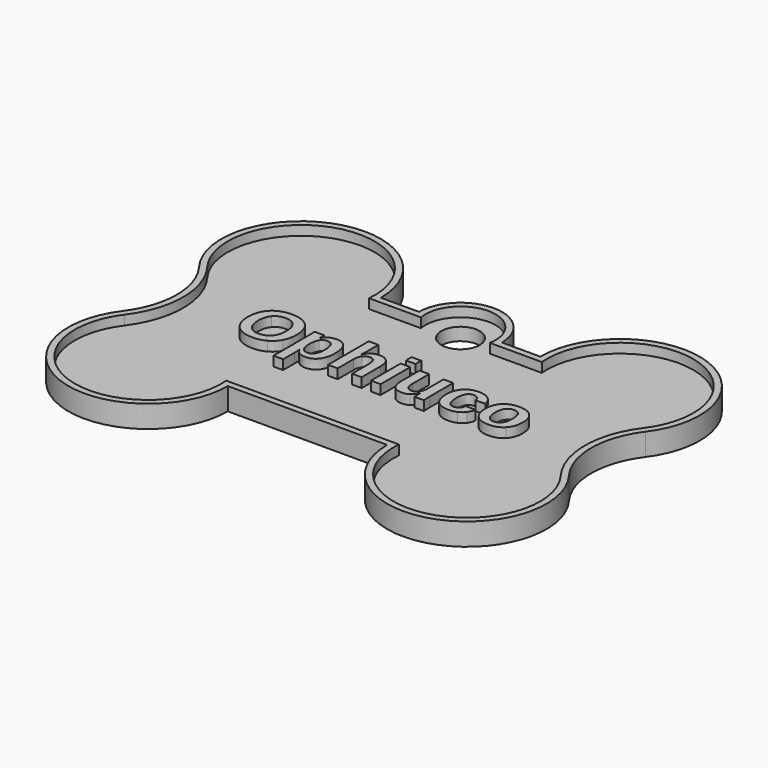
from build123d import *

# Parameters (mm, degrees)
F0_R     = 3
F1_DEPTH = 3.5
F2_W     = 1.5111876076
F2_H     = 5.8192771084
F2_H_2   = 1.1135972461
F3_DEPTH = 1.5


with BuildPart() as f1:
    # F0 (on Top) → F1 (new body)
    with BuildSketch(Plane.XY):
        with BuildLine():
            Line((28.5, 30), (22.5, 30))
            ThreePointArc((22.5, 30), (6.0471529248, 41.8585412256), (0, 22.5))
            ThreePointArc((0, 22.5), (2.5, 15), (0, 7.5))
            ThreePointArc((0, 7.5), (6.0471529248, -11.8585412256), (22.5, 0))
            Line((22.5, 0), (47.5, 0))
            ThreePointArc((47.5, 0), (63.9528470752, -11.8585412256), (70, 7.5))
            ThreePointArc((70, 7.5), (67.5, 15), (70, 22.5))
            ThreePointArc((70, 22.5), (63.9528470752, 41.8585412256), (47.5, 30))
            Line((47.5, 30), (41.5, 30))
            ThreePointArc((41.5, 30), (35, 36.5), (28.5, 30))
        make_face()
        with Locations((35, 30)):
            Circle(F0_R, mode=Mode.SUBTRACT)
    extrude(amount=F1_DEPTH)

    # F2 (on face) → F3 (cut)
    with BuildSketch(Plane.XY.offset(3.5)):
        with BuildLine():
            Line((21.4564392374, 1), (48.5435607626, 1))
            ThreePointArc((48.5435607626, 1), (63.1583824195, -11.0577855148), (69.2, 6.9))
            ThreePointArc((69.2, 6.9), (66.5, 15), (69.2, 23.1))
            ThreePointArc((69.2, 23.1), (63.1583824195, 41.0577855148), (48.5435607626, 29))
            Line((48.5435607626, 29), (40.4083269132, 29))
            ThreePointArc((40.4083269132, 29), (35, 35.5), (29.5916730868, 29))
            Line((29.5916730868, 29), (21.4564392374, 29))
            ThreePointArc((21.4564392374, 29), (6.8416175805, 41.0577855148), (0.8, 23.1))
            ThreePointArc((0.8, 23.1), (3.5, 15), (0.8, 6.9))
            ThreePointArc((0.8, 6.9), (6.8416175805, -11.0577855148), (21.4564392374, 1))
        make_face()
        with BuildLine():
            add(Edge.make_bspline(
                [(26.7857142857, 17.2297762478), (27.3450946644, 16.4475043029), (27.3450946644, 15.0051635112)],
                knots=[0, 0, 0, 1, 1, 1], degree=2))
            add(Edge.make_bspline(
                [(27.3450946644, 15.0051635112), (27.3450946644, 13.5473321859), (26.7616179002, 12.7538726334)],
                knots=[0, 0, 0, 1, 1, 1], degree=2))
            add(Edge.make_bspline(
                [(26.7616179002, 12.7538726334), (26.178141136, 11.9604130809), (25.1127366609, 11.9604130809)],
                knots=[0, 0, 0, 1, 1, 1], degree=2))
            add(Edge.make_bspline(
                [(25.1127366609, 11.9604130809), (24.5, 11.9604130809), (24.0456110155, 12.2271944923)],
                knots=[0, 0, 0, 1, 1, 1], degree=2))
            add(Edge.make_bspline(
                [(24.0456110155, 12.2271944923), (23.591222031, 12.4939759036), (23.3485370052, 12.9948364888)],
                knots=[0, 0, 0, 1, 1, 1], degree=2))
            Line((23.3485370052, 12.9948364888), (23.3158347676, 12.9948364888))
            add(Edge.make_bspline(
                [(23.3158347676, 12.9948364888), (23.3485370052, 12.8330464716), (23.3485370052, 12.0154905336)],
                knots=[0, 0, 0, 1, 1, 1], degree=2))
            Line((23.3485370052, 12.0154905336), (23.3485370052, 9.7831325301))
            Line((23.3485370052, 9.7831325301), (21.8373493976, 9.7831325301))
            Line((21.8373493976, 9.7831325301), (21.8373493976, 16.5490533563))
            add(Edge.make_bspline(
                [(21.8373493976, 16.5490533563), (21.8373493976, 17.3717728055), (21.7943201377, 17.8881239243)],
                knots=[0, 0, 0, 1, 1, 1], degree=2))
            Line((21.7943201377, 17.8881239243), (23.2624784854, 17.8881239243))
            add(Edge.make_bspline(
                [(23.2624784854, 17.8881239243), (23.2900172117, 17.7917383821), (23.3089500861, 17.5068846816)],
                knots=[0, 0, 0, 1, 1, 1], degree=2))
            add(Edge.make_bspline(
                [(23.3089500861, 17.5068846816), (23.3278829604, 17.2220309811), (23.3278829604, 16.9414802065)],
                knots=[0, 0, 0, 1, 1, 1], degree=2))
            Line((23.3278829604, 16.9414802065), (23.3485370052, 16.9414802065))
            add(Edge.make_bspline(
                [(23.3485370052, 16.9414802065), (23.8597246127, 18.0120481928), (25.2091222031, 18.0120481928)],
                knots=[0, 0, 0, 1, 1, 1], degree=2))
            add(Edge.make_bspline(
                [(25.2091222031, 18.0120481928), (26.2263339071, 18.0120481928), (26.7857142857, 17.2297762478)],
                knots=[0, 0, 0, 1, 1, 1], degree=2))
        make_face(mode=Mode.SUBTRACT)
        with Locations((36.0490533563, 14.9784853701)):
            Rectangle(F2_W, F2_H, mode=Mode.SUBTRACT)
        with BuildLine():
            Line((38.2676419966, 17.8881239243), (39.7788296041, 17.8881239243))
            Line((39.7788296041, 17.8881239243), (39.7788296041, 14.6230636833))
            add(Edge.make_bspline(
                [(39.7788296041, 14.6230636833), (39.7788296041, 13.091222031), (40.8115318417, 13.091222031)],
                knots=[0, 0, 0, 1, 1, 1], degree=2))
            add(Edge.make_bspline(
                [(40.8115318417, 13.091222031), (41.3605851979, 13.091222031), (41.6962134251, 13.5619621343)],
                knots=[0, 0, 0, 1, 1, 1], degree=2))
            add(Edge.make_bspline(
                [(41.6962134251, 13.5619621343), (42.0318416523, 14.0327022375), (42.0318416523, 14.769363167)],
                knots=[0, 0, 0, 1, 1, 1], degree=2))
            Line((42.0318416523, 14.769363167), (42.0318416523, 17.8881239243))
            Line((42.0318416523, 17.8881239243), (43.5447504303, 17.8881239243))
            Line((43.5447504303, 17.8881239243), (43.5447504303, 13.3700516351))
            add(Edge.make_bspline(
                [(43.5447504303, 13.3700516351), (43.5447504303, 12.6282271945), (43.5877796902, 12.0688468158)],
                knots=[0, 0, 0, 1, 1, 1], degree=2))
            Line((43.5877796902, 12.0688468158), (42.1454388985, 12.0688468158))
            add(Edge.make_bspline(
                [(42.1454388985, 12.0688468158), (42.0817555938, 12.843373494), (42.0817555938, 13.2254733219)],
                knots=[0, 0, 0, 1, 1, 1], degree=2))
            Line((42.0817555938, 13.2254733219), (42.0542168675, 13.2254733219))
            add(Edge.make_bspline(
                [(42.0542168675, 13.2254733219), (41.7530120482, 12.5645438898), (41.2874354561, 12.2624784854)],
                knots=[0, 0, 0, 1, 1, 1], degree=2))
            add(Edge.make_bspline(
                [(41.2874354561, 12.2624784854), (40.821858864, 11.9604130809), (40.1815834768, 11.9604130809)],
                knots=[0, 0, 0, 1, 1, 1], degree=2))
            add(Edge.make_bspline(
                [(40.1815834768, 11.9604130809), (39.2573149742, 11.9604130809), (38.7624784854, 12.5283993115)],
                knots=[0, 0, 0, 1, 1, 1], degree=2))
            add(Edge.make_bspline(
                [(38.7624784854, 12.5283993115), (38.2676419966, 13.0963855422), (38.2676419966, 14.1927710843)],
                knots=[0, 0, 0, 1, 1, 1], degree=2))
            Line((38.2676419966, 14.1927710843), (38.2676419966, 17.8881239243))
        make_face(mode=Mode.SUBTRACT)
        with BuildLine():
            add(Edge.make_bspline(
                [(48.7771084337, 12.2160068847), (48.2125645439, 11.9604130809), (47.5068846816, 11.9604130809)],
                knots=[0, 0, 0, 1, 1, 1], degree=2))
            add(Edge.make_bspline(
                [(47.5068846816, 11.9604130809), (46.1850258176, 11.9604130809), (45.4638554217, 12.7487091222)],
                knots=[0, 0, 0, 1, 1, 1], degree=2))
            add(Edge.make_bspline(
                [(45.4638554217, 12.7487091222), (44.7426850258, 13.5370051635), (44.7426850258, 14.9466437177)],
                knots=[0, 0, 0, 1, 1, 1], degree=2))
            add(Edge.make_bspline(
                [(44.7426850258, 14.9466437177), (44.7426850258, 16.3872633391), (45.4690189329, 17.1919104991)],
                knots=[0, 0, 0, 1, 1, 1], degree=2))
            add(Edge.make_bspline(
                [(45.4690189329, 17.1919104991), (46.1953528399, 17.9965576592), (47.5292598967, 17.9965576592)],
                knots=[0, 0, 0, 1, 1, 1], degree=2))
            add(Edge.make_bspline(
                [(47.5292598967, 17.9965576592), (48.5567986231, 17.9965576592), (49.2289156627, 17.4802065404)],
                knots=[0, 0, 0, 1, 1, 1], degree=2))
            add(Edge.make_bspline(
                [(49.2289156627, 17.4802065404), (49.9010327022, 16.9638554217), (50.0731497418, 16.0550774527)],
                knots=[0, 0, 0, 1, 1, 1], degree=2))
            Line((50.0731497418, 16.0550774527), (48.5516351119, 15.9793459552))
            add(Edge.make_bspline(
                [(48.5516351119, 15.9793459552), (48.4862306368, 16.4251290878), (48.2280550775, 16.6919104991)],
                knots=[0, 0, 0, 1, 1, 1], degree=2))
            add(Edge.make_bspline(
                [(48.2280550775, 16.6919104991), (47.9698795181, 16.9586919105), (47.4965576592, 16.9586919105)],
                knots=[0, 0, 0, 1, 1, 1], degree=2))
            add(Edge.make_bspline(
                [(47.4965576592, 16.9586919105), (46.3296041308, 16.9586919105), (46.3296041308, 15.0051635112)],
                knots=[0, 0, 0, 1, 1, 1], degree=2))
            add(Edge.make_bspline(
                [(46.3296041308, 15.0051635112), (46.3296041308, 12.9948364888), (47.5189328744, 12.9948364888)],
                knots=[0, 0, 0, 1, 1, 1], degree=2))
            add(Edge.make_bspline(
                [(47.5189328744, 12.9948364888), (47.9492254733, 12.9948364888), (48.239242685, 13.2659208262)],
                knots=[0, 0, 0, 1, 1, 1], degree=2))
            add(Edge.make_bspline(
                [(48.239242685, 13.2659208262), (48.5292598967, 13.5370051635), (48.599827883, 14.0757314974)],
                knots=[0, 0, 0, 1, 1, 1], degree=2))
            Line((48.599827883, 14.0757314974), (50.1161790017, 14.0051635112))
            add(Edge.make_bspline(
                [(50.1161790017, 14.0051635112), (50.0352839931, 13.4079173838), (49.6884681583, 12.9397590361)],
                knots=[0, 0, 0, 1, 1, 1], degree=2))
            add(Edge.make_bspline(
                [(49.6884681583, 12.9397590361), (49.3416523236, 12.4716006885), (48.7771084337, 12.2160068847)],
                knots=[0, 0, 0, 1, 1, 1], degree=2))
        make_face(mode=Mode.SUBTRACT)
        with BuildLine():
            add(Edge.make_bspline(
                [(55.9862306368, 17.2194492255), (56.7358003442, 16.4423407917), (56.7358003442, 14.9845094664)],
                knots=[0, 0, 0, 1, 1, 1], degree=2))
            add(Edge.make_bspline(
                [(56.7358003442, 14.9845094664), (56.7358003442, 13.569707401), (55.9509466437, 12.765060241)],
                knots=[0, 0, 0, 1, 1, 1], degree=2))
            add(Edge.make_bspline(
                [(55.9509466437, 12.765060241), (55.1660929432, 11.9604130809), (53.7788296041, 11.9604130809)],
                knots=[0, 0, 0, 1, 1, 1], degree=2))
            add(Edge.make_bspline(
                [(53.7788296041, 11.9604130809), (52.417383821, 11.9604130809), (51.6428571429, 12.7676419966)],
                knots=[0, 0, 0, 1, 1, 1], degree=2))
            add(Edge.make_bspline(
                [(51.6428571429, 12.7676419966), (50.8683304647, 13.5748709122), (50.8683304647, 14.9845094664)],
                knots=[0, 0, 0, 1, 1, 1], degree=2))
            add(Edge.make_bspline(
                [(50.8683304647, 14.9845094664), (50.8683304647, 16.3872633391), (51.6428571429, 17.1919104991)],
                knots=[0, 0, 0, 1, 1, 1], degree=2))
            add(Edge.make_bspline(
                [(51.6428571429, 17.1919104991), (52.417383821, 17.9965576592), (53.8098106713, 17.9965576592)],
                knots=[0, 0, 0, 1, 1, 1], degree=2))
            add(Edge.make_bspline(
                [(53.8098106713, 17.9965576592), (55.2366609294, 17.9965576592), (55.9862306368, 17.2194492255)],
                knots=[0, 0, 0, 1, 1, 1], degree=2))
        make_face(mode=Mode.SUBTRACT)
        with BuildLine():
            add(Edge.make_bspline(
                [(19.591222031, 18.7280550775), (20.6049913941, 17.6953528399), (20.6049913941, 15.8932874355)],
                knots=[0, 0, 0, 1, 1, 1], degree=2))
            add(Edge.make_bspline(
                [(20.6049913941, 15.8932874355), (20.6049913941, 14.7091222031), (20.1376936317, 13.8115318417)],
                knots=[0, 0, 0, 1, 1, 1], degree=2))
            add(Edge.make_bspline(
                [(20.1376936317, 13.8115318417), (19.6703958692, 12.9139414802), (18.7986230637, 12.4371772806)],
                knots=[0, 0, 0, 1, 1, 1], degree=2))
            add(Edge.make_bspline(
                [(18.7986230637, 12.4371772806), (17.9268502582, 11.9604130809), (16.765060241, 11.9604130809)],
                knots=[0, 0, 0, 1, 1, 1], degree=2))
            add(Edge.make_bspline(
                [(16.765060241, 11.9604130809), (14.9802065404, 11.9604130809), (13.9664371773, 13.0120481928)],
                knots=[0, 0, 0, 1, 1, 1], degree=2))
            add(Edge.make_bspline(
                [(13.9664371773, 13.0120481928), (12.9526678141, 14.0636833046), (12.9526678141, 15.8932874355)],
                knots=[0, 0, 0, 1, 1, 1], degree=2))
            add(Edge.make_bspline(
                [(12.9526678141, 15.8932874355), (12.9526678141, 17.7160068847), (13.9638554217, 18.7383820998)],
                knots=[0, 0, 0, 1, 1, 1], degree=2))
            add(Edge.make_bspline(
                [(13.9638554217, 18.7383820998), (14.9750430293, 19.760757315), (16.7762478485, 19.760757315)],
                knots=[0, 0, 0, 1, 1, 1], degree=2))
            add(Edge.make_bspline(
                [(16.7762478485, 19.760757315), (18.5774526678, 19.760757315), (19.591222031, 18.7280550775)],
                knots=[0, 0, 0, 1, 1, 1], degree=2))
        make_face(mode=Mode.SUBTRACT)
        with BuildLine():
            Line((30.0335628227, 16.7263339071), (30.0559380379, 16.7263339071))
            add(Edge.make_bspline(
                [(30.0559380379, 16.7263339071), (30.3623063683, 17.3941480207), (30.8244406196, 17.6953528399)],
                knots=[0, 0, 0, 1, 1, 1], degree=2))
            add(Edge.make_bspline(
                [(30.8244406196, 17.6953528399), (31.2865748709, 17.9965576592), (31.9268502582, 17.9965576592)],
                knots=[0, 0, 0, 1, 1, 1], degree=2))
            add(Edge.make_bspline(
                [(31.9268502582, 17.9965576592), (32.8528399312, 17.9965576592), (33.34767642, 17.425989673)],
                knots=[0, 0, 0, 1, 1, 1], degree=2))
            add(Edge.make_bspline(
                [(33.34767642, 17.425989673), (33.8425129088, 16.8554216867), (33.8425129088, 15.7590361446)],
                knots=[0, 0, 0, 1, 1, 1], degree=2))
            Line((33.8425129088, 15.7590361446), (33.8425129088, 12.0688468158))
            Line((33.8425129088, 12.0688468158), (32.3364888124, 12.0688468158))
            Line((32.3364888124, 12.0688468158), (32.3364888124, 15.3287435456))
            add(Edge.make_bspline(
                [(32.3364888124, 15.3287435456), (32.3364888124, 16.8605851979), (31.2969018933, 16.8605851979)],
                knots=[0, 0, 0, 1, 1, 1], degree=2))
            add(Edge.make_bspline(
                [(31.2969018933, 16.8605851979), (30.7495697074, 16.8605851979), (30.413080895, 16.3907056799)],
                knots=[0, 0, 0, 1, 1, 1], degree=2))
            add(Edge.make_bspline(
                [(30.413080895, 16.3907056799), (30.0765920826, 15.9208261618), (30.0765920826, 15.182444062)],
                knots=[0, 0, 0, 1, 1, 1], degree=2))
            Line((30.0765920826, 15.182444062), (30.0765920826, 12.0688468158))
            Line((30.0765920826, 12.0688468158), (28.565404475, 12.0688468158))
            Line((28.565404475, 12.0688468158), (28.565404475, 20.0516351119))
            Line((28.565404475, 20.0516351119), (30.0765920826, 20.0516351119))
            Line((30.0765920826, 20.0516351119), (30.0765920826, 17.8726333907))
            add(Edge.make_bspline(
                [(30.0765920826, 17.8726333907), (30.0765920826, 17.2857142857), (30.0335628227, 16.7263339071)],
                knots=[0, 0, 0, 1, 1, 1], degree=2))
        make_face(mode=Mode.SUBTRACT)
        with Locations((36.0490533563, 19.4948364888)):
            Rectangle(F2_W, F2_H_2, mode=Mode.SUBTRACT)
        with BuildLine():
            add(Edge.make_bspline(
                [(18.408777969, 13.908777969), (18.987091222, 14.6075731497), (18.987091222, 15.8932874355)],
                knots=[0, 0, 0, 1, 1, 1], degree=2))
            add(Edge.make_bspline(
                [(18.987091222, 15.8932874355), (18.987091222, 17.1187607573), (18.4061962134, 17.8158347676)],
                knots=[0, 0, 0, 1, 1, 1], degree=2))
            add(Edge.make_bspline(
                [(18.4061962134, 17.8158347676), (17.8253012048, 18.512908778), (16.7753872633, 18.512908778)],
                knots=[0, 0, 0, 1, 1, 1], degree=2))
            add(Edge.make_bspline(
                [(16.7753872633, 18.512908778), (15.7117039587, 18.512908778), (15.1308089501, 17.821858864)],
                knots=[0, 0, 0, 1, 1, 1], degree=2))
            add(Edge.make_bspline(
                [(15.1308089501, 17.821858864), (14.5499139415, 17.1308089501), (14.5499139415, 15.8932874355)],
                knots=[0, 0, 0, 1, 1, 1], degree=2))
            add(Edge.make_bspline(
                [(14.5499139415, 15.8932874355), (14.5499139415, 14.6454388985), (15.1437177281, 13.9277108434)],
                knots=[0, 0, 0, 1, 1, 1], degree=2))
            add(Edge.make_bspline(
                [(15.1437177281, 13.9277108434), (15.7375215146, 13.2099827883), (16.765060241, 13.2099827883)],
                knots=[0, 0, 0, 1, 1, 1], degree=2))
            add(Edge.make_bspline(
                [(16.765060241, 13.2099827883), (17.830464716, 13.2099827883), (18.408777969, 13.908777969)],
                knots=[0, 0, 0, 1, 1, 1], degree=2))
        make_face()
        with BuildLine():
            add(Edge.make_bspline(
                [(24.5585197935, 12.9948364888), (25.7685025818, 12.9948364888), (25.7685025818, 15.0051635112)],
                knots=[0, 0, 0, 1, 1, 1], degree=2))
            add(Edge.make_bspline(
                [(25.7685025818, 15.0051635112), (25.7685025818, 16.9638554217), (24.5688468158, 16.9638554217)],
                knots=[0, 0, 0, 1, 1, 1], degree=2))
            add(Edge.make_bspline(
                [(24.5688468158, 16.9638554217), (23.9664371773, 16.9638554217), (23.6471600688, 16.4363166954)],
                knots=[0, 0, 0, 1, 1, 1], degree=2))
            add(Edge.make_bspline(
                [(23.6471600688, 16.4363166954), (23.3278829604, 15.908777969), (23.3278829604, 14.9621342513)],
                knots=[0, 0, 0, 1, 1, 1], degree=2))
            add(Edge.make_bspline(
                [(23.3278829604, 14.9621342513), (23.3278829604, 14.0206540448), (23.6471600688, 13.5077452668)],
                knots=[0, 0, 0, 1, 1, 1], degree=2))
            add(Edge.make_bspline(
                [(23.6471600688, 13.5077452668), (23.9664371773, 12.9948364888), (24.5585197935, 12.9948364888)],
                knots=[0, 0, 0, 1, 1, 1], degree=2))
        make_face()
        with BuildLine():
            add(Edge.make_bspline(
                [(53.7616179002, 12.9948364888), (55.1557659208, 12.9948364888), (55.1557659208, 14.9845094664)],
                knots=[0, 0, 0, 1, 1, 1], degree=2))
            add(Edge.make_bspline(
                [(55.1557659208, 14.9845094664), (55.1557659208, 16.0223752151), (54.8166953528, 16.4905335628)],
                knots=[0, 0, 0, 1, 1, 1], degree=2))
            add(Edge.make_bspline(
                [(54.8166953528, 16.4905335628), (54.4776247849, 16.9586919105), (53.8321858864, 16.9586919105)],
                knots=[0, 0, 0, 1, 1, 1], degree=2))
            add(Edge.make_bspline(
                [(53.8321858864, 16.9586919105), (52.4552495697, 16.9586919105), (52.4552495697, 14.9845094664)],
                knots=[0, 0, 0, 1, 1, 1], degree=2))
            add(Edge.make_bspline(
                [(52.4552495697, 14.9845094664), (52.4552495697, 14.0103270224), (52.7917383821, 13.5025817556)],
                knots=[0, 0, 0, 1, 1, 1], degree=2))
            add(Edge.make_bspline(
                [(52.7917383821, 13.5025817556), (53.1282271945, 12.9948364888), (53.7616179002, 12.9948364888)],
                knots=[0, 0, 0, 1, 1, 1], degree=2))
        make_face()
    extrude(amount=-F3_DEPTH, mode=Mode.SUBTRACT)


solid = f1.part
